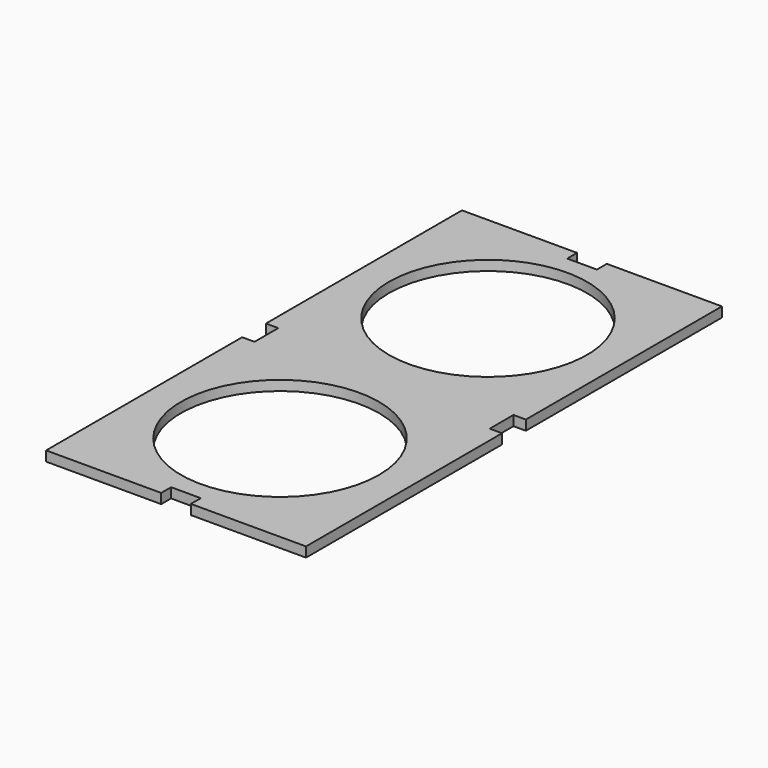
from build123d import *

# Parameters (mm, degrees)
F1_DEPTH = 12.7


with BuildPart() as f1:
    # F0 (on Top) → F1 (new body)
    with BuildSketch(Plane.XY):
        with BuildLine():
            Line((166.6875, -333.375), (166.6875, -166.6875))
            Line((166.6875, -166.6875), (127, -166.6875))
            ThreePointArc((127, -166.6875), (0, -293.6875), (-127, -166.6875))
            Line((-127, -166.6875), (-166.6875, -166.6875))
            Line((-166.6875, -166.6875), (-166.6875, -333.375))
            Line((-166.6875, -333.375), (-19.05, -333.375))
            Line((-19.05, -333.375), (-19.05, -317.5))
            Line((-19.05, -317.5), (19.05, -317.5))
            Line((19.05, -317.5), (19.05, -333.375))
            Line((19.05, -333.375), (166.6875, -333.375))
        make_face()
        with BuildLine():
            Line((127, 166.6875), (166.6875, 166.6875))
            Line((166.6875, 166.6875), (166.6875, 333.375))
            Line((166.6875, 333.375), (19.05, 333.375))
            Line((19.05, 333.375), (19.05, 317.5))
            Line((19.05, 317.5), (-19.05, 317.5))
            Line((-19.05, 317.5), (-19.05, 333.375))
            Line((-19.05, 333.375), (-166.6875, 333.375))
            Line((-166.6875, 333.375), (-166.6875, 166.6875))
            Line((-166.6875, 166.6875), (-127, 166.6875))
            ThreePointArc((-127, 166.6875), (0, 293.6875), (127, 166.6875))
        make_face()
        with BuildLine():
            Line((127, -166.6875), (166.6875, -166.6875))
            Line((166.6875, -166.6875), (166.6875, -19.05))
            Line((166.6875, -19.05), (150.8125, -19.05))
            Line((150.8125, -19.05), (150.8125, 19.05))
            Line((150.8125, 19.05), (166.6875, 19.05))
            Line((166.6875, 19.05), (166.6875, 166.6875))
            Line((166.6875, 166.6875), (127, 166.6875))
            ThreePointArc((127, 166.6875), (0, 39.6875), (-127, 166.6875))
            Line((-127, 166.6875), (-166.6875, 166.6875))
            Line((-166.6875, 166.6875), (-166.6875, 19.05))
            Line((-166.6875, 19.05), (-150.8125, 19.05))
            Line((-150.8125, 19.05), (-150.8125, -19.05))
            Line((-150.8125, -19.05), (-166.6875, -19.05))
            Line((-166.6875, -19.05), (-166.6875, -166.6875))
            Line((-166.6875, -166.6875), (-127, -166.6875))
            ThreePointArc((-127, -166.6875), (0, -39.6875), (127, -166.6875))
        make_face()
    extrude(amount=F1_DEPTH)


solid = f1.part
